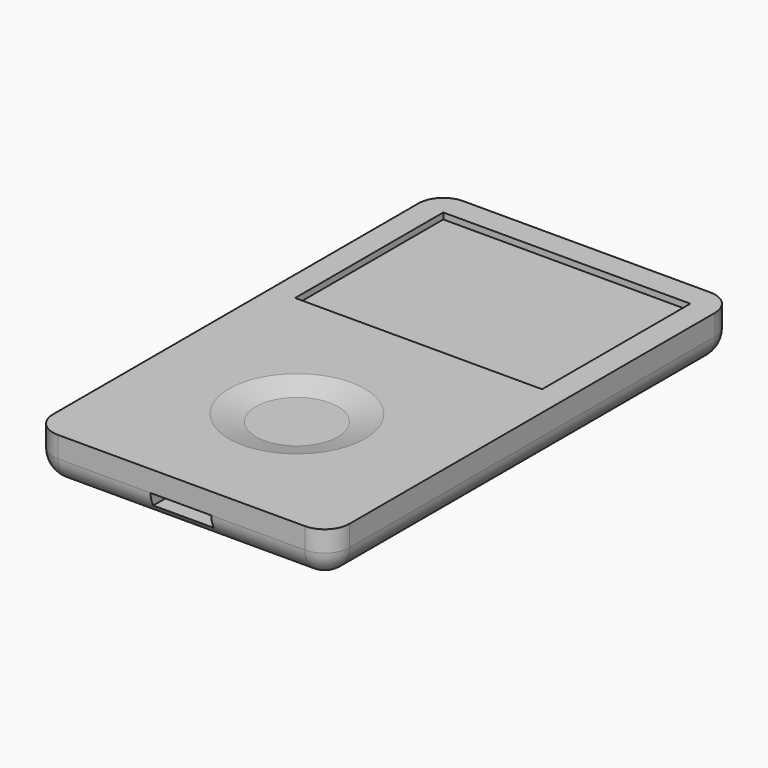
from build123d import *

# Parameters (mm, degrees)
F0_R         = 17.78
F0_W         = 50.8
F0_H         = 38.1
F0_R_2       = 7.62
F1_DEPTH     = 9.398
F2_W         = 12.4930366991
F2_H         = 2.54
F3_DEPTH     = 6.35
F4_W         = 9.7033483908
F4_H         = 2.4660443887
F4_R         = 1.3462908927
F4_R_2       = 1.087736237
F5_DEPTH     = 3.1496
F6_DEPTH     = 0.2286
F7_R         = 0.3066051224
F8_T1_DEPTH  = 93.98
F8_T3_DEPTH  = 50.8
F8_T6_ANGLE  = 90
F8_T8_ANGLE  = 90
F8_T10_ANGLE = 90
F8_T12_ANGLE = 90
F9_START     = 8.128
F9_DEPTH     = 1.524


# Not quite as in the source:
# - a fillet or chamfer that OpenCascade refuses, or shapes differently, is made with other operations: its cross-section is extruded or revolved along the edge and cut away or added


with BuildPart() as f1:
    # F0 (on Top) → F1 (new body)
    with BuildSketch(Plane.XY):
        with BuildLine():
            Line((25.4, 52.07), (-25.4, 52.07))
            ThreePointArc((-25.4, 52.07), (-28.9921024484, 50.5821024484), (-30.48, 46.99))
            Line((-30.48, 46.99), (-30.48, -46.99))
            ThreePointArc((-30.48, -46.99), (-28.9921024484, -50.5821024484), (-25.4, -52.07))
            Line((-25.4, -52.07), (25.4, -52.07))
            ThreePointArc((25.4, -52.07), (28.9921024484, -50.5821024484), (30.48, -46.99))
            Line((30.48, -46.99), (30.48, 46.99))
            ThreePointArc((30.48, 46.99), (28.9921024484, 50.5821024484), (25.4, 52.07))
        make_face()
        with Locations((0, -21.59)):
            Circle(F0_R, mode=Mode.SUBTRACT)
        with Locations((0, 27.94)):
            Rectangle(F0_W, F0_H, mode=Mode.SUBTRACT)
        with Locations((0, -21.59)):
            Circle(F0_R)
        with Locations((0, -21.59)):
            Circle(F0_R_2, mode=Mode.SUBTRACT)
        with Locations((0, -21.59)):
            Circle(F0_R_2)
        with Locations((0, 27.94)):
            Rectangle(F0_W, F0_H)
    extrude(amount=F1_DEPTH)

    # F2 (on face) → F3 (cut)
    with BuildSketch(Plane.XZ.offset(52.07)):
        with Locations((-0.0956295989, 3.81)):
            Rectangle(F2_W, F2_H)
    extrude(amount=-F3_DEPTH, mode=Mode.SUBTRACT)

    # F4 (on face) → F5 (cut)
    with BuildSketch(Plane(origin=(0, 52.07, 0), x_dir=(-1, 0, 0), z_dir=(0, 1, 0))):
        with Locations((-17.8750143386, 7.5830221944)):
            Rectangle(F4_W, F4_H)
        with Locations((18.9737091073, 7.7977091073)):
            Circle(F4_R)
        with Locations((18.9737091073, 7.7977091073)):
            Circle(F4_R_2, mode=Mode.SUBTRACT)
    extrude(amount=-F5_DEPTH, mode=Mode.SUBTRACT)

    # F6 (add): a face of the model
    f6_faces = [f1.faces().sort_by_distance(p)[0] for p in [
        (-18.9737091073, 52.07, 7.7977091073),
    ]]
    extrude(f6_faces, amount=F6_DEPTH)

    # F7
    f7_edges = [f1.edges().sort_by_distance(p)[0] for p in [
        (-17.885973, 52.2986, 7.797709),
    ]]
    fillet(f7_edges, radius=F7_R)

    # F8: fillet of radius 5.08 on 1 edges, made by hand

    # F8_s2 → F8_t1 (cut)
    with BuildSketch(Plane.XZ.offset(-46.99)):
        with BuildLine():
            ThreePointArc((-25.4, 0), (-28.9921024484, 1.4878975516), (-30.48, 5.08))
            Line((-30.48, 5.08), (-30.48, 0))
            Line((-30.48, 0), (-25.4, 0))
        make_face()
        with BuildLine():
            ThreePointArc((25.4, 0), (28.9921024484, 1.4878975516), (30.48, 5.08))
            Line((30.48, 5.08), (30.48, 0))
            Line((30.48, 0), (25.4, 0))
        make_face()
    extrude(amount=F8_T1_DEPTH, mode=Mode.SUBTRACT)

    # F8_s4 → F8_t3 (cut)
    with BuildSketch(Plane.YZ.offset(-25.4)):
        with BuildLine():
            ThreePointArc((-46.99, 0), (-50.5821024484, 1.4878975516), (-52.07, 5.08))
            Line((-52.07, 5.08), (-52.07, 0))
            Line((-52.07, 0), (-46.99, 0))
        make_face()
        with BuildLine():
            ThreePointArc((52.07, 5.08), (50.5821024484, 1.4878975516), (46.99, 0))
            Line((46.99, 0), (52.07, 0))
            Line((52.07, 0), (52.07, 5.08))
        make_face()
    extrude(amount=F8_T3_DEPTH, mode=Mode.SUBTRACT)

    # F8_s5 → F8_t6 (revolve, cut)
    with BuildSketch(Plane.XZ.offset(46.99)):
        with BuildLine():
            ThreePointArc((-25.4, 0), (-28.9921024484, 1.4878975516), (-30.48, 5.08))
            Line((-30.48, 5.08), (-30.48, 0))
            Line((-30.48, 0), (-25.4, 0))
        make_face()
    revolve(axis=Axis((-25.4, -46.99, 0), (0, 0, 1)), revolution_arc=F8_T6_ANGLE, mode=Mode.SUBTRACT)

    # F8_s7 → F8_t8 (revolve, cut)
    with BuildSketch(Plane.YZ.offset(25.4)):
        with BuildLine():
            ThreePointArc((-46.99, 0), (-50.5821024484, 1.4878975516), (-52.07, 5.08))
            Line((-52.07, 5.08), (-52.07, 0))
            Line((-52.07, 0), (-46.99, 0))
        make_face()
    revolve(axis=Axis((25.4, -46.99, 0), (0, 0, 1)), revolution_arc=F8_T8_ANGLE, mode=Mode.SUBTRACT)

    # F8_s9 → F8_t10 (revolve, cut)
    with BuildSketch(Plane.XZ.offset(-46.99)):
        with BuildLine():
            ThreePointArc((30.48, 5.08), (28.9921024484, 1.4878975516), (25.4, 0))
            Line((25.4, 0), (30.48, 0))
            Line((30.48, 0), (30.48, 5.08))
        make_face()
    revolve(axis=Axis((25.4, 46.99, 0), (0, 0, 1)), revolution_arc=F8_T10_ANGLE, mode=Mode.SUBTRACT)

    # F8_s11 → F8_t12 (revolve, cut)
    with BuildSketch(Plane.YZ.offset(-25.4)):
        with BuildLine():
            ThreePointArc((46.99, 0), (50.5821024484, 1.4878975516), (52.07, 5.08))
            Line((52.07, 5.08), (52.07, 0))
            Line((52.07, 0), (46.99, 0))
        make_face()
    revolve(axis=Axis((-25.4, 46.99, 0), (0, 0, 1)), revolution_arc=F8_T12_ANGLE, mode=Mode.SUBTRACT)

    # F0 (on Top) → F9 (cut)
    with BuildSketch(Plane.XY.offset(F9_START)):
        with Locations((0, 27.94)):
            Rectangle(F0_W, F0_H)
    extrude(amount=F9_DEPTH, mode=Mode.SUBTRACT)

    # F10 (on Right) → F11 (revolve, cut)
    with BuildSketch(Plane.YZ):
        Polygon((-7.623700425, 9.6026211977), (-22.3824381828, 9.6026211977), (-22.3824381828, 7.986061275), (-13.9484070241, 7.986061275), align=None)
    revolve(axis=Axis((0, -22.3824381828, 9.8022762686), (0, 0, 1)), mode=Mode.SUBTRACT)


solid = f1.part
